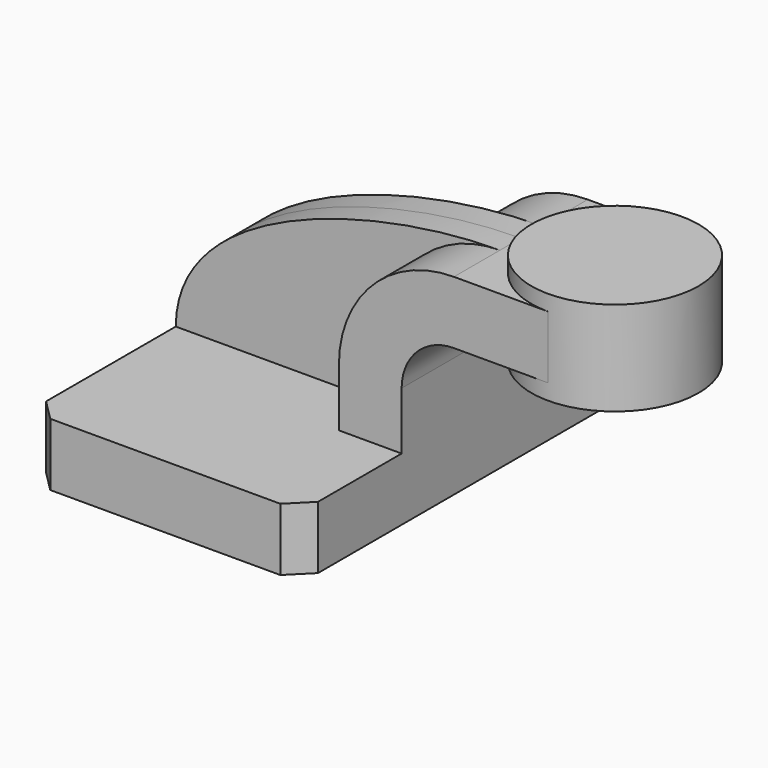
from build123d import *

# Parameters (mm, degrees)
F1_DEPTH = 63.5
F0_W     = 25.4
F0_H     = 19.05
F2_DEPTH = 25.4
F3_DEPTH = 7.9375
F5_SIZE  = 6.35


# Not quite as in the source:
# - a feature names something its author has since deleted; it is built from what else it names


with BuildPart() as f1:
    # F0 (on Front) → F1 (new body, symmetric)
    with BuildSketch(Plane.XZ):
        Polygon((-41.275, 9.525), (-41.275, -9.525), (41.275, -9.525), (41.275, 9.525), (22.225, 9.525), align=None)
    extrude(amount=F1_DEPTH, both=True)

    # F0 (on Front) → F2 (join, symmetric)
    with BuildSketch(Plane.XZ):
        with BuildLine():
            Line((22.225, 9.525), (41.275, 9.525))
            Line((41.275, 9.525), (41.275, 27.0002))
            ThreePointArc((41.275, 27.0002), (45.9246798487, 38.2255201513), (57.15, 42.8752))
            Line((57.15, 42.8752), (60.325, 42.8752))
            Line((60.325, 42.8752), (60.325, 61.9252))
            Line((60.325, 61.9252), (57.15, 61.9252))
            ThreePointArc((57.15, 61.9252), (32.4542956671, 51.6959043329), (22.225, 27.0002))
            Line((22.225, 27.0002), (22.225, 9.525))
        make_face()
        with Locations((73.025, 52.4002)):
            Rectangle(F0_W, F0_H)
    extrude(amount=F2_DEPTH, both=True)

    # F0 (on Front) → F3 (join, symmetric)
    with BuildSketch(Plane.XZ):
        with BuildLine():
            add(Edge.make_bspline(
                [(-41.275, 9.525), (-41.0928055644, 45.868396759), (20.8572410047, 62.0456375182), (57.15, 61.9252)],
                knots=[0, 0, 0, 0, 111.5045361635, 111.5045361635, 111.5045361635, 111.5045361635], degree=3))
            Line((-41.275, 9.525), (22.225, 9.525))
            Line((22.225, 9.525), (22.225, 27.0002))
            ThreePointArc((22.225, 27.0002), (32.4542956671, 51.6959043329), (57.15, 61.9252))
        make_face()
    extrude(amount=F3_DEPTH, both=True)

    # F0 (on Front) → F4 (revolve)
    with BuildSketch(Plane.XZ):
        Polygon((85.725, 66.675), (85.725, 61.9252), (85.725, 42.8752), (85.725, 38.1), (111.125, 38.1), (111.125, 66.675), align=None)
    revolve(axis=Axis((85.725, 0, 52.3875), (0, 0, -1)))

    # F5
    f5_edges = [f1.edges().sort_by_distance(p)[0] for p in [
        (41.275, -63.5, 0),
        (-41.275, -63.5, 0),
        (41.275, 63.5, 0),
        (-41.275, 63.5, 0),
    ]]
    chamfer(f5_edges, length=F5_SIZE)


solid = f1.part
